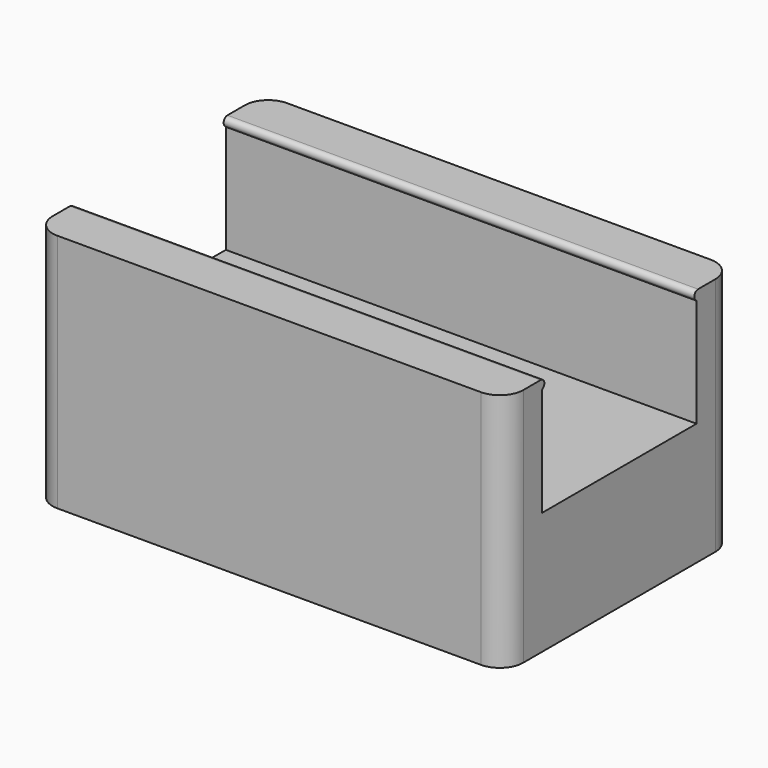
from build123d import *

# Parameters (mm, degrees)
F0_W         = 100
F0_H         = 10
F1_DEPTH     = 51
F2_DEPTH     = 26
F3_DEPTH     = 29
F4_R         = 5
F5_W         = 100
F5_H         = 3
F6_DEPTH     = 2
F7_T4_DEPTH  = 115.4300979278
F8_W         = 100
F8_H         = 3
F9_DEPTH     = 2
F10_T4_DEPTH = 115.4300979278
F11_R        = 1


# Not quite as in the source:
# - a fillet or chamfer that OpenCascade refuses, or shapes differently, is made with other operations: its cross-section is extruded or revolved along the edge and cut away or added


with BuildPart() as f1:
    # F0 (on Top) → F1 (new body)
    with BuildSketch(Plane.XY):
        with Locations((50, -5)):
            Rectangle(F0_W, F0_H)
    extrude(amount=F1_DEPTH)



with BuildPart() as f1b:
    # F0 (on Top) → F1, piece 2 (new body)
    with BuildSketch(Plane.XY):
        with Locations((50, -56)):
            Rectangle(F0_W, F0_H)
    extrude(amount=F1_DEPTH)


with BuildPart() as f1_1:
    add(f1.part)

    add(f1b.part)  # F2 merges F1b
    # F0 (on Top) → F2 (join)
    with BuildSketch(Plane.XY):
        with Locations((50, -5)):
            Rectangle(F0_W, F0_H)
        with BuildLine():
            Line((100, -10), (0, -10))
            Line((0, -10), (0, -30.5))
            Line((0, -30.5), (46, -30.5))
            ThreePointArc((46, -30.5), (50, -26.5), (54, -30.5))
            Line((54, -30.5), (100, -30.5))
            Line((100, -30.5), (100, -10))
        make_face()
        with BuildLine():
            Line((46, -30.5), (0, -30.5))
            Line((0, -30.5), (0, -51))
            Line((0, -51), (100, -51))
            Line((100, -51), (100, -30.5))
            Line((100, -30.5), (54, -30.5))
            ThreePointArc((54, -30.5), (50, -34.5), (46, -30.5))
        make_face()
        with Locations((50, -56)):
            Rectangle(F0_W, F0_H)
        with BuildLine():
            ThreePointArc((54, -30.5), (50, -26.5), (46, -30.5))
            Line((46, -30.5), (49, -30.5))
            ThreePointArc((49, -30.5), (50, -29.5), (51, -30.5))
            Line((51, -30.5), (54, -30.5))
        make_face()
        with BuildLine():
            Line((49, -30.5), (46, -30.5))
            ThreePointArc((46, -30.5), (50, -34.5), (54, -30.5))
            Line((54, -30.5), (51, -30.5))
            ThreePointArc((51, -30.5), (50, -31.5), (49, -30.5))
        make_face()
    extrude(amount=F2_DEPTH)

    # F0 (on Top) → F3 (join)
    with BuildSketch(Plane.XY):
        with BuildLine():
            ThreePointArc((54, -30.5), (50, -26.5), (46, -30.5))
            Line((46, -30.5), (49, -30.5))
            ThreePointArc((49, -30.5), (50, -29.5), (51, -30.5))
            Line((51, -30.5), (54, -30.5))
        make_face()
        with BuildLine():
            Line((49, -30.5), (46, -30.5))
            ThreePointArc((46, -30.5), (50, -34.5), (54, -30.5))
            Line((54, -30.5), (51, -30.5))
            ThreePointArc((51, -30.5), (50, -31.5), (49, -30.5))
        make_face()
    extrude(amount=F3_DEPTH)

    # F4
    f4_edges = [f1_1.edges().sort_by_distance(p)[0] for p in [
        (100, 0, 25.5),
        (0, 0, 25.5),
        (100, -61, 25.5),
        (0, -61, 25.5),
    ]]
    fillet(f4_edges, radius=F4_R)

    # F5 (on face) → F6 (join)
    with BuildSketch(Plane.XY.offset(51)):
        with Locations((50, -11.5)):
            Rectangle(F5_W, F5_H)
    extrude(amount=-F6_DEPTH)

    # F7: chamfer of 3 on 1 edges, made by hand


with BuildPart() as f7_tool2:
    # F7_s3 → F7_t4 (new body)
    with BuildSketch(Plane.YZ.offset(-7.7150489639)):
        Polygon((-10, 49), (-13, 52), (-13, 49), align=None)
    extrude(amount=F7_T4_DEPTH)

    split(bisect_by=Plane.XZ.offset(10), keep=Keep.TOP)


with BuildPart() as f1_2:
    add(f1_1.part)

    # F7_t1: cut F7_tool2
    add(f7_tool2.part, mode=Mode.SUBTRACT)

    # F8 (on face) → F9 (join)
    with BuildSketch(Plane.XY.offset(51)):
        with Locations((50, -49.5)):
            Rectangle(F8_W, F8_H)
    extrude(amount=-F9_DEPTH)

    # F10: chamfer of 3 on 1 edges, made by hand


with BuildPart() as f10_tool2:
    # F10_s3 → F10_t4 (new body)
    with BuildSketch(Plane.YZ.offset(107.7150489639)):
        Polygon((-51, 49), (-48, 52), (-48, 49), align=None)
    extrude(amount=-F10_T4_DEPTH)

    split(bisect_by=Plane.XZ.offset(51), keep=Keep.BOTTOM)


with BuildPart() as f1_3:
    add(f1_2.part)

    # F10_t1: cut F10_tool2
    add(f10_tool2.part, mode=Mode.SUBTRACT)

    # F11
    f11_edges = [f1_3.edges().sort_by_distance(p)[0] for p in [
        (50, -12, 51),
        (50, -49, 51),
    ]]
    fillet(f11_edges, radius=F11_R)


solid = f1_3.part
